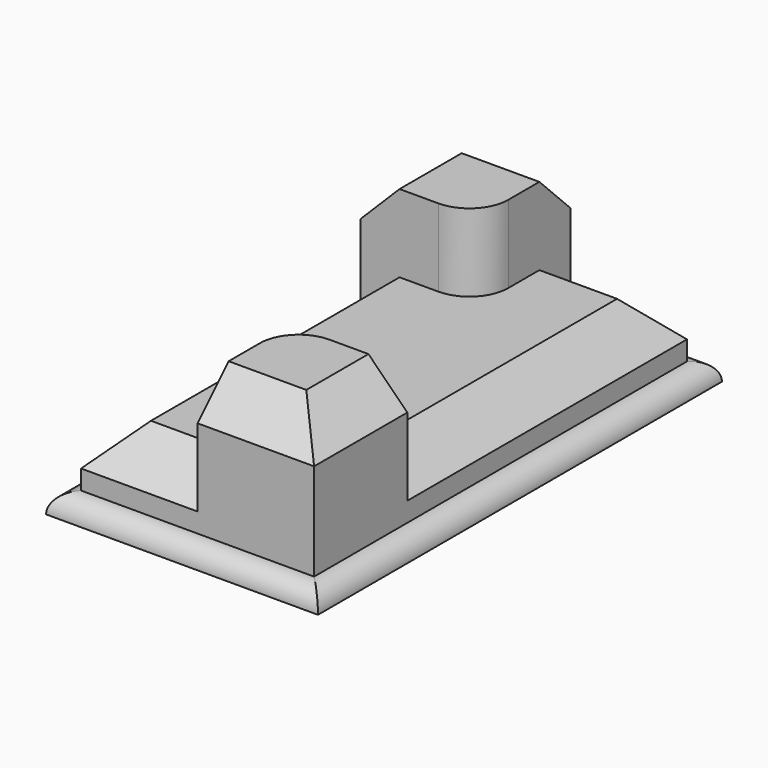
from build123d import *

# Parameters (mm, degrees)
F0_W     = 88.9
F0_H     = 165.1
F1_DEPTH = 6.35
F2_DEPTH = 25.4
F3_DEPTH = 50.8
F4_R     = 6.34999
F5_SIZE  = 12.7


# Not quite as in the source:
# - a fillet or chamfer is up to 0.001 mm smaller than in the source, because OpenCascade refuses the exact size


with BuildPart() as f1:
    # F0 (on Top) → F1 (new body)
    with BuildSketch(Plane.XY):
        with Locations((-1.8205753744, 3.0884221945)):
            Rectangle(F0_W, F0_H)
        Polygon((-39.9205753744, 41.1884221945), (-39.9205753744, 79.2884221945), (-1.8205753744, 79.2884221945), (36.2794246256, 79.2884221945), (36.2794246256, -35.0115778055), (36.2794246256, -73.1115778055), (-1.8205753744, -73.1115778055), (-39.9205753744, -73.1115778055), align=None, mode=Mode.SUBTRACT)
    extrude(amount=F1_DEPTH)

    # F0 (on Top) → F2 (join)
    with BuildSketch(Plane.XY):
        with BuildLine():
            Line((36.2794246256, 79.2884221945), (-1.8205753744, 79.2884221945))
            Line((-1.8205753744, 79.2884221945), (-1.8205753744, 53.8884221945))
            ThreePointArc((-1.8205753744, 53.8884221945), (-5.5403192533, 44.9081660734), (-14.5205753744, 41.1884221945))
            Line((-14.5205753744, 41.1884221945), (-39.9205753744, 41.1884221945))
            Line((-39.9205753744, 41.1884221945), (-39.9205753744, -73.1115778055))
            Line((-39.9205753744, -73.1115778055), (-1.8205753744, -73.1115778055))
            Line((-1.8205753744, -73.1115778055), (-1.8205753744, -47.7115778055))
            ThreePointArc((-1.8205753744, -47.7115778055), (1.8991685046, -38.7313216844), (10.8794246256, -35.0115778055))
            Line((10.8794246256, -35.0115778055), (36.2794246256, -35.0115778055))
            Line((36.2794246256, -35.0115778055), (36.2794246256, 79.2884221945))
        make_face()
    extrude(amount=F2_DEPTH)

    # F0 (on Top) → F3 (join)
    with BuildSketch(Plane.XY):
        with BuildLine():
            Line((-1.8205753744, 79.2884221945), (-39.9205753744, 79.2884221945))
            Line((-39.9205753744, 79.2884221945), (-39.9205753744, 41.1884221945))
            Line((-39.9205753744, 41.1884221945), (-14.5205753744, 41.1884221945))
            ThreePointArc((-14.5205753744, 41.1884221945), (-5.5403192533, 44.9081660734), (-1.8205753744, 53.8884221945))
            Line((-1.8205753744, 53.8884221945), (-1.8205753744, 79.2884221945))
        make_face()
        with BuildLine():
            Line((36.2794246256, -73.1115778055), (36.2794246256, -35.0115778055))
            Line((36.2794246256, -35.0115778055), (10.8794246256, -35.0115778055))
            ThreePointArc((10.8794246256, -35.0115778055), (1.8991685046, -38.7313216844), (-1.8205753744, -47.7115778055))
            Line((-1.8205753744, -47.7115778055), (-1.8205753744, -73.1115778055))
            Line((-1.8205753744, -73.1115778055), (36.2794246256, -73.1115778055))
        make_face()
    extrude(amount=F3_DEPTH)

    # F4 (radius 6.35 in the source; OpenCascade refuses exactly that, so slightly less here)
    f4_edges = [f1.edges().sort_by_distance(p)[0] for p in [
        (-46.270575, 3.088422, 6.35),
        (-1.820575, -79.461578, 6.35),
        (42.629425, 3.088422, 6.35),
        (-1.820575, 85.638422, 6.35),
    ]]
    fillet(f4_edges, radius=F4_R)

    # F5
    f5_edges = [f1.edges().sort_by_distance(p)[0] for p in [
        (17.229425, -73.111578, 50.8),
        (36.279425, -54.061578, 50.8),
        (-39.920575, 60.238422, 50.8),
        (-20.870575, 79.288422, 50.8),
        (-39.920575, -15.961578, 25.4),
        (-20.870575, -73.111578, 25.4),
        (36.279425, 22.138422, 25.4),
        (17.229425, 79.288422, 25.4),
    ]]
    chamfer(f5_edges, length=F5_SIZE)


solid = f1.part
